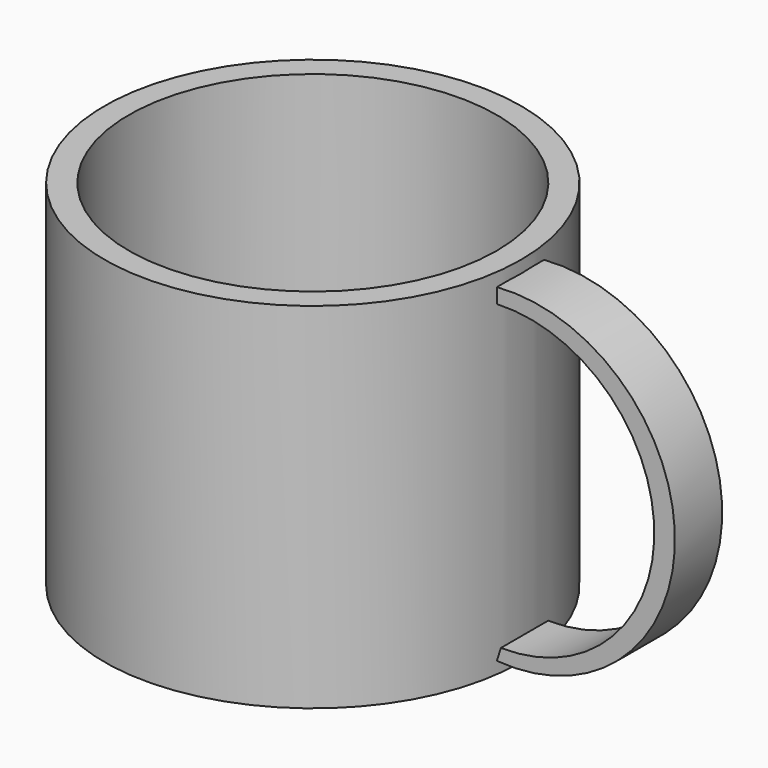
from build123d import *

# Parameters (mm, degrees)
F0_R          = 44.803850357
F0_R_2        = 39.5649031507
F1_DEPTH      = 76.2
F0_R_3        = 39.4553703488
F2_DEPTH      = 0.254
F4_DEPTH      = 6.35
F4_DEPTH_BACK = 6.35


# Not quite as in the source:
# - the program builds the solid bodies; features that only make, move or delete a surface that nothing else refers to are left out


with BuildPart() as f1:
    # F0 (on Top) → F1 (new body)
    with BuildSketch(Plane.XY):
        Circle(F0_R)
        Circle(F0_R_2, mode=Mode.SUBTRACT)
    extrude(amount=F1_DEPTH)

    # F3 (on Front) → F4 (join, two sides)
    with BuildSketch(Plane.XZ) as f4_sk:
        with BuildLine():
            ThreePointArc((44.6730293334, 70.3529790044), (78.5293989005, 38.3747792802), (45.5318614841, 5.5110980757))
            Line((45.5318614841, 5.5110980757), (44.6730293334, 2.7786104474))
            ThreePointArc((44.6730293334, 2.7786104474), (82.974605628, 38.1732090609), (44.6730293334, 73.5678076744))
            Line((44.6730293334, 73.5678076744), (44.6730293334, 70.3529790044))
        make_face()
    extrude(amount=F4_DEPTH)
    extrude(f4_sk.sketch, amount=-F4_DEPTH_BACK)


with BuildPart() as f2:
    # F0 (on Top) → F2 (new body)
    with BuildSketch(Plane.XY):
        Circle(F0_R_3)
    extrude(amount=-F2_DEPTH)


solid = Compound([f1.part, f2.part])
